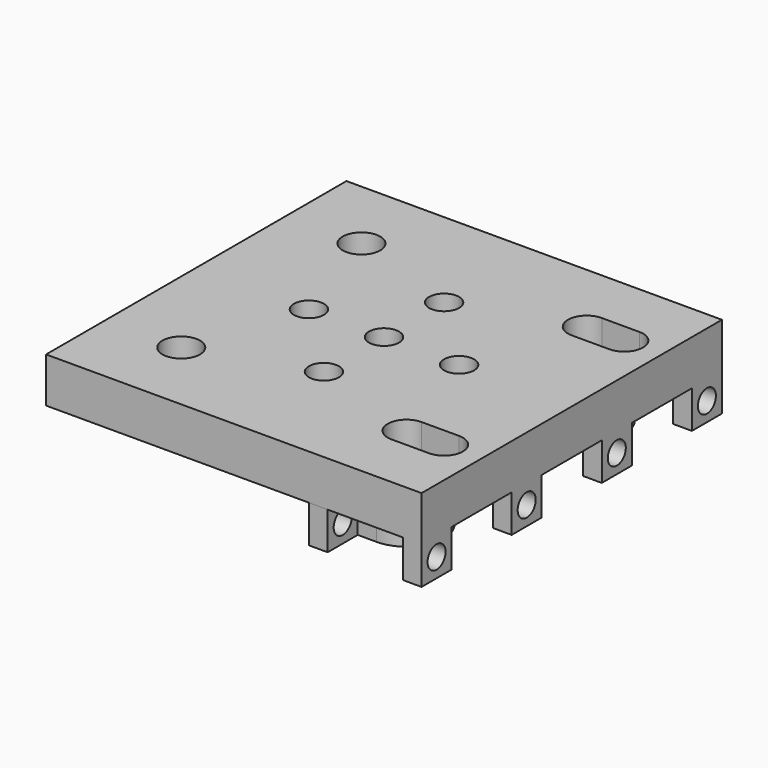
from build123d import *

# Parameters (mm, degrees)
F0_R             = 2
F1_DEPTH         = 6
F2_W             = 2.5
F2_H             = 5
F3_DEPTH         = 5
F5_DEPTH         = 5
F8_D             = 3
F8_DEPTH         = 40
F8_TIP           = 0.9012909285
F8_2_D           = 3
F8_2_DEPTH       = 40
F8_2_TIP         = 0.9012909285
F8_ON_F6_D       = 3
F8_ON_F6_DEPTH   = 40
F8_ON_F6_TIP     = 0.9012909285
F8_ON_F6_2_D     = 3
F8_ON_F6_2_DEPTH = 40
F8_ON_F6_2_TIP   = 0.9012909285


with BuildPart() as f1:
    # F0 (on Top) → F1 (new body)
    with BuildSketch(Plane.XY):
        Polygon((25, 15), (25, 25), (-25, 25), (-25, 15), (-25, -15), (-25, -25), (25, -25), (25, -15), align=None)
        with BuildLine():
            ThreePointArc((-12.5, -15), (-15, -17.5), (-17.5, -15))
            ThreePointArc((-17.5, -15), (-15, -12.5), (-12.5, -15))
        make_face(mode=Mode.SUBTRACT)
        with BuildLine():
            ThreePointArc((20, -12.5), (21.767766953, -13.232233047), (22.5, -15))
            ThreePointArc((22.5, -15), (21.767766953, -16.767766953), (20, -17.5))
            Line((20, -17.5), (15, -17.5))
            ThreePointArc((15, -17.5), (12.5, -15), (15, -12.5))
            Line((15, -12.5), (20, -12.5))
        make_face(mode=Mode.SUBTRACT)
        with Locations((0, -10)):
            Circle(F0_R, mode=Mode.SUBTRACT)
        with Locations((-10, 0)):
            Circle(F0_R, mode=Mode.SUBTRACT)
        with BuildLine():
            ThreePointArc((-12.5, 15), (-15, 12.5), (-17.5, 15))
            ThreePointArc((-17.5, 15), (-15, 17.5), (-12.5, 15))
        make_face(mode=Mode.SUBTRACT)
        Circle(F0_R, mode=Mode.SUBTRACT)
        with Locations((10, 0)):
            Circle(F0_R, mode=Mode.SUBTRACT)
        with Locations((0, 10)):
            Circle(F0_R, mode=Mode.SUBTRACT)
        with BuildLine():
            ThreePointArc((20, 17.5), (21.767766953, 16.767766953), (22.5, 15))
            ThreePointArc((22.5, 15), (21.767766953, 13.232233047), (20, 12.5))
            Line((20, 12.5), (15, 12.5))
            ThreePointArc((15, 12.5), (12.5, 15), (15, 17.5))
            Line((15, 17.5), (20, 17.5))
        make_face(mode=Mode.SUBTRACT)
    extrude(amount=F1_DEPTH)

    # F2 (on face) → F3 (join)
    with BuildSketch(Plane(origin=(0, 0, 0), x_dir=(1, 0, 0), z_dir=(0, 0, -1))):
        with Locations((23.75, 22.5)):
            Rectangle(F2_W, F2_H)
        with Locations((23.75, 7.5)):
            Rectangle(F2_W, F2_H)
        with Locations((23.75, -7.5)):
            Rectangle(F2_W, F2_H)
        with Locations((23.75, -22.5)):
            Rectangle(F2_W, F2_H)
    extrude(amount=F3_DEPTH)

    # F8
    with Locations(Plane(origin=(10, 0, 0), x_dir=(0, -1, 0), z_dir=(-1, 0, 0))):
        with Locations((-7.5, -2.5), (-22.5, -2.5)):
            Hole(F8_D / 2, depth=F8_DEPTH)
            with Locations((0, 0, -(F8_DEPTH + F8_TIP / 2))):  # 118° drill point
                Cone(0, F8_D / 2, F8_TIP, mode=Mode.SUBTRACT)

    # F8 on F6
    with Locations(Plane(origin=(10, 0, 0), x_dir=(0, -1, 0), z_dir=(-1, 0, 0))):
        with Locations((7.5, -2.5), (22.5, -2.5)):
            Hole(F8_ON_F6_D / 2, depth=F8_ON_F6_DEPTH)
            with Locations((0, 0, -(F8_ON_F6_DEPTH + F8_ON_F6_TIP / 2))):  # 118° drill point
                Cone(0, F8_ON_F6_D / 2, F8_ON_F6_TIP, mode=Mode.SUBTRACT)


with BuildPart() as f5:
    # F4 (on face) → F5 (new body)
    with BuildSketch(Plane(origin=(0, 0, 0), x_dir=(1, 0, 0), z_dir=(0, 0, -1))):
        with BuildLine():
            Line((12.5, 19.3301270189), (12.5, 20))
            Line((12.5, 20), (12.5, 25))
            Line((12.5, 25), (10, 25))
            Line((10, 25), (10, 15))
            ThreePointArc((10, 15), (10.6698729811, 17.5), (12.5, 19.3301270189))
        make_face()
        with BuildLine():
            Line((15, 20), (12.5, 20))
            Line((12.5, 20), (12.5, 19.3301270189))
            ThreePointArc((12.5, 19.3301270189), (13.7059047745, 19.8296291314), (15, 20))
        make_face()
        with BuildLine():
            ThreePointArc((15, 20), (13.7059047745, 19.8296291314), (12.5, 19.3301270189))
            Line((12.5, 19.3301270189), (12.5, 15))
            ThreePointArc((12.5, 15), (13.232233047, 16.767766953), (15, 17.5))
            Line((15, 17.5), (19.3301270189, 17.5))
            ThreePointArc((19.3301270189, 17.5), (17.5, 19.3301270189), (15, 20))
        make_face()
        with BuildLine():
            Line((12.5, 15), (12.5, 19.3301270189))
            ThreePointArc((12.5, 19.3301270189), (10.6698729811, 17.5), (10, 15))
            ThreePointArc((10, 15), (10.6698729811, 12.5), (12.5, 10.6698729811))
            Line((12.5, 10.6698729811), (12.5, 15))
        make_face()
        with BuildLine():
            ThreePointArc((15, 12.5), (13.232233047, 13.232233047), (12.5, 15))
            Line((12.5, 15), (12.5, 10.6698729811))
            ThreePointArc((12.5, 10.6698729811), (13.7059047745, 10.1703708686), (15, 10))
            ThreePointArc((15, 10), (17.5, 10.6698729811), (19.3301270189, 12.5))
            Line((19.3301270189, 12.5), (15, 12.5))
        make_face()
        with BuildLine():
            ThreePointArc((12.5, 10.6698729811), (10.6698729811, 12.5), (10, 15))
            Line((10, 15), (10, 5))
            Line((10, 5), (12.5, 5))
            Line((12.5, 5), (12.5, 10))
            Line((12.5, 10), (12.5, 10.6698729811))
        make_face()
        with BuildLine():
            ThreePointArc((20, 15), (19.8296291314, 16.2940952255), (19.3301270189, 17.5))
            Line((19.3301270189, 17.5), (15, 17.5))
            ThreePointArc((15, 17.5), (16.767766953, 16.767766953), (17.5, 15))
            ThreePointArc((17.5, 15), (16.767766953, 13.232233047), (15, 12.5))
            Line((15, 12.5), (19.3301270189, 12.5))
            ThreePointArc((19.3301270189, 12.5), (19.8296291314, 13.7059047745), (20, 15))
        make_face()
        with BuildLine():
            ThreePointArc((15, 10), (13.7059047745, 10.1703708686), (12.5, 10.6698729811))
            Line((12.5, 10.6698729811), (12.5, 10))
            Line((12.5, 10), (15, 10))
        make_face()
    extrude(amount=F5_DEPTH)

    # F8 on F6#2
    with Locations(Plane(origin=(10, 0, 0), x_dir=(0, -1, 0), z_dir=(-1, 0, 0))):
        with Locations((7.5, -2.5), (22.5, -2.5)):
            Hole(F8_ON_F6_2_D / 2, depth=F8_ON_F6_2_DEPTH)
            with Locations((0, 0, -(F8_ON_F6_2_DEPTH + F8_ON_F6_2_TIP / 2))):  # 118° drill point
                Cone(0, F8_ON_F6_2_D / 2, F8_ON_F6_2_TIP, mode=Mode.SUBTRACT)


with BuildPart() as f5b:
    # F4 (on face) → F5, piece 2 (new body)
    with BuildSketch(Plane(origin=(0, 0, 0), x_dir=(1, 0, 0), z_dir=(0, 0, -1))):
        with BuildLine():
            Line((10, -15), (10, -25))
            Line((10, -25), (12.5, -25))
            Line((12.5, -25), (12.5, -20))
            Line((12.5, -20), (12.5, -19.3301270189))
            ThreePointArc((12.5, -19.3301270189), (10.6698729811, -17.5), (10, -15))
        make_face()
        with BuildLine():
            Line((12.5, -10), (12.5, -5))
            Line((12.5, -5), (10, -5))
            Line((10, -5), (10, -15))
            ThreePointArc((10, -15), (10.6698729811, -12.5), (12.5, -10.6698729811))
            Line((12.5, -10.6698729811), (12.5, -10))
        make_face()
        with BuildLine():
            ThreePointArc((12.5, -10.6698729811), (10.6698729811, -12.5), (10, -15))
            ThreePointArc((10, -15), (10.6698729811, -17.5), (12.5, -19.3301270189))
            Line((12.5, -19.3301270189), (12.5, -15))
            Line((12.5, -15), (12.5, -10.6698729811))
        make_face()
        with BuildLine():
            Line((15, -10), (12.5, -10))
            Line((12.5, -10), (12.5, -10.6698729811))
            ThreePointArc((12.5, -10.6698729811), (13.7059047745, -10.1703708686), (15, -10))
        make_face()
        with BuildLine():
            ThreePointArc((15, -10), (13.7059047745, -10.1703708686), (12.5, -10.6698729811))
            Line((12.5, -10.6698729811), (12.5, -15))
            ThreePointArc((12.5, -15), (13.232233047, -13.232233047), (15, -12.5))
            Line((15, -12.5), (19.3301270189, -12.5))
            ThreePointArc((19.3301270189, -12.5), (17.5, -10.6698729811), (15, -10))
        make_face()
        with BuildLine():
            ThreePointArc((15, -20), (13.7059047745, -19.8296291314), (12.5, -19.3301270189))
            Line((12.5, -19.3301270189), (12.5, -20))
            Line((12.5, -20), (15, -20))
        make_face()
        with BuildLine():
            Line((12.5, -15), (12.5, -19.3301270189))
            ThreePointArc((12.5, -19.3301270189), (13.7059047745, -19.8296291314), (15, -20))
            ThreePointArc((15, -20), (17.5, -19.3301270189), (19.3301270189, -17.5))
            Line((19.3301270189, -17.5), (15, -17.5))
            ThreePointArc((15, -17.5), (13.232233047, -16.767766953), (12.5, -15))
        make_face()
        with BuildLine():
            ThreePointArc((20, -15), (19.8296291314, -13.7059047745), (19.3301270189, -12.5))
            Line((19.3301270189, -12.5), (15, -12.5))
            ThreePointArc((15, -12.5), (16.767766953, -13.232233047), (17.5, -15))
            ThreePointArc((17.5, -15), (16.767766953, -16.767766953), (15, -17.5))
            Line((15, -17.5), (19.3301270189, -17.5))
            ThreePointArc((19.3301270189, -17.5), (19.8296291314, -16.2940952255), (20, -15))
        make_face()
    extrude(amount=F5_DEPTH)

    # F8#2
    with Locations(Plane(origin=(10, 0, 0), x_dir=(0, -1, 0), z_dir=(-1, 0, 0))):
        with Locations((-7.5, -2.5), (-22.5, -2.5)):
            Hole(F8_2_D / 2, depth=F8_2_DEPTH)
            with Locations((0, 0, -(F8_2_DEPTH + F8_2_TIP / 2))):  # 118° drill point
                Cone(0, F8_2_D / 2, F8_2_TIP, mode=Mode.SUBTRACT)


solid = Compound([f1.part, f5.part, f5b.part])
